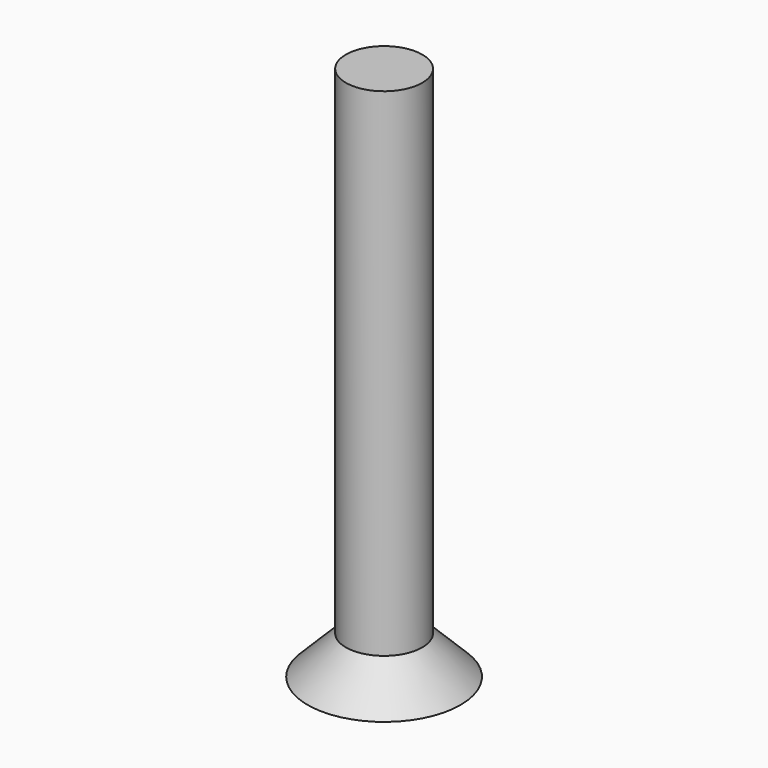
from build123d import *

# Parameters (mm, degrees)
F0_R     = 5
F1_DEPTH = 2.5
F2_SIZE  = 2.49999
F3_DEPTH = 32.5


# Not quite as in the source:
# - a fillet or chamfer is up to 0.001 mm smaller than in the source, because OpenCascade refuses the exact size


with BuildPart() as f1:
    # F0 (on Top) → F1 (new body)
    with BuildSketch(Plane.XY):
        Circle(F0_R)
    extrude(amount=F1_DEPTH)

    # F2 (size 2.5 in the source; OpenCascade refuses exactly that, so slightly less here)
    f2_edges = [f1.edges().sort_by_distance(p)[0] for p in [
        (-5, 0, 2.5),
    ]]
    chamfer(f2_edges, length=F2_SIZE)

    # F3 (add): a face of the model
    f3_faces = [f1.faces().sort_by_distance(p)[0] for p in [
        (0, 0, 2.5),
    ]]
    extrude(f3_faces, amount=F3_DEPTH)


solid = f1.part
